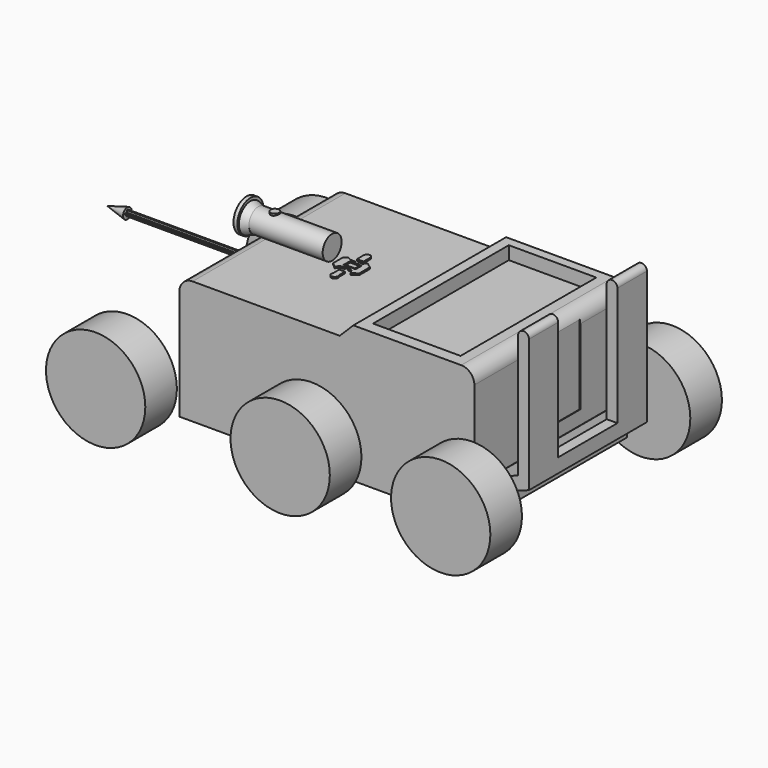
from build123d import *

# Parameters (mm, degrees)
F0_W           = 112
F0_H           = 52
F1_DEPTH       = 36.25
F1_DEPTH_BACK  = 36.25
F2_W           = 62.7835113555
F2_H           = 8.2989688963
F3_DEPTH       = 40
F3_DEPTH_BACK  = 40
F4_SIZE        = 5
F5_R           = 5
F8_DEPTH       = 0.6
F9_W           = 3.3755060285
F9_H           = 2.0101326518
F10_DEPTH      = 0.6
F12_R          = 18.8548205179
F13_DEPTH      = 15
F19_R          = 18.8548205179
F20_DEPTH      = 15
F24_DEPTH      = 28
F24_DEPTH_BACK = 28
F26_W          = 28.1342324962
F26_H          = 48.9349166028
F27_DEPTH      = 25
F29_R          = 4.5035590708
F30_DEPTH      = 28
F32_R          = 6.2065419795
F33_DEPTH      = 1.5
F36_R          = 4.4303853292
F37_DEPTH      = 25
F38_R          = 1.617072427
F39_DEPTH      = 9.3
F40_W          = 33.2386381924
F40_H          = 64.4318200648
F41_DEPTH      = 25
F42_R          = 1.0614733058
F43_DEPTH      = 80
F45_DEPTH      = 90


# Not quite as in the source:
# - the program builds the solid bodies; features that only make, move or delete a surface that nothing else refers to are left out


with BuildPart() as f1:
    # F0 (on Front) → F1 (new body, two sides)
    with BuildSketch(Plane.XZ) as f1_sk:
        Rectangle(F0_W, F0_H)
    extrude(amount=F1_DEPTH)
    extrude(f1_sk.sketch, amount=-F1_DEPTH_BACK)

    # F2 (on Front) → F3 (cut, two sides)
    with BuildSketch(Plane.XZ) as f3_sk:
        with Locations((-26.3402080163, 24.9871136621)):
            Rectangle(F2_W, F2_H)
    extrude(amount=-F3_DEPTH, mode=Mode.SUBTRACT)
    extrude(f3_sk.sketch, amount=F3_DEPTH_BACK, mode=Mode.SUBTRACT)

    # F4
    f4_edges = [f1.edges().sort_by_distance(p)[0] for p in [
        (5.051548, 0, 26),
    ]]
    chamfer(f4_edges, length=F4_SIZE)

    # F5
    f5_edges = [f1.edges().sort_by_distance(p)[0] for p in [
        (56, 0, 26),
        (-56, 0, 20.837629),
    ]]
    fillet(f5_edges, radius=F5_R)

    # F23 (on Front) → F24 (join, two sides)
    with BuildSketch(Plane.XZ) as f24_sk:
        with BuildLine():
            Line((66.0493522882, -9.3606118894), (56.0777671635, -12.9401576556))
            ThreePointArc((56.0777671635, -12.9401576556), (52.810402565, -15.2911024559), (56.0777671635, -17.6420472562))
            Line((56.0777671635, -17.6420472562), (70.1072718896, -12.9401576556))
            Line((70.1072718896, -12.9401576556), (70.1072718896, 37.5393816017))
            ThreePointArc((70.1072718896, 37.5393816017), (67.878123137, 39.5765729642), (66.0493522882, 37.1734812074))
            Line((66.0493522882, 37.1734812074), (66.0493522882, -9.3606118894))
        make_face()
    extrude(amount=F24_DEPTH)
    extrude(f24_sk.sketch, amount=-F24_DEPTH_BACK)

    # F26 (on offset) → F27 (cut)
    with BuildSketch(Plane.YZ.offset(55.8)):
        with Locations((-0.0549908727, 16.8750025332)):
            Rectangle(F26_W, F26_H)
    extrude(amount=F27_DEPTH, mode=Mode.SUBTRACT)

    # F29 (on offset) → F30 (join)
    with BuildSketch(Plane.YZ.offset(-27)):
        with Locations((0, 25.3125000745)):
            Circle(F29_R)
    extrude(amount=-F30_DEPTH)

    # F38 (on offset) → F39 (join)
    with BuildSketch(Plane.XY.offset(21)):
        with Locations((-48.7517826259, 0)):
            Circle(F38_R)
    extrude(amount=F39_DEPTH)

    # F40 (on offset) → F41 (cut)
    with BuildSketch(Plane.XY.offset(21)):
        with Locations((30.5095855147, 0.5113650113)):
            Rectangle(F40_W, F40_H)
    extrude(amount=F41_DEPTH, mode=Mode.SUBTRACT)

    # F42 (on offset) → F43 (join)
    with BuildSketch(Plane.YZ.offset(-27)):
        with Locations((0, 11.5056820214)):
            Circle(F42_R)
    extrude(amount=-F43_DEPTH)

    # F44 (on offset) → F45 (cut)
    with BuildSketch(Plane.YZ.offset(-58)):
        Polygon((-0.9458741988, 10.3932730854), (-0.3025215992, 10.4609942064), (-0.3025215992, 11.1382082105), (-1.1828994611, 11.1382082105), align=None)
        Polygon((1.2212089496, 11.1382082105), (0.3069706145, 11.1382082105), (0.3069706145, 10.4609942064), (0.8487420273, 10.3594120592), align=None)
        Polygon((-1.3505744282, 11.729169637), (-0.2593955433, 11.729169637), (-0.2593955433, 12.6839512959), (-1.2141767656, 12.4306418002), (-1.2921184534, 12.0214503258), (-1.3505744282, 11.865567416), align=None)
        Polygon((1.1240632739, 12.7813778818), (0.3056792775, 12.7813778818), (0.3056792775, 11.7486547679), (1.2604609365, 11.7486547679), align=None)
    extrude(amount=-F45_DEPTH, mode=Mode.SUBTRACT)

    # F46 (on Front) → F47 (revolve)
    with BuildSketch(Plane.XZ):
        Polygon((-104.7758087516, 9.3221208081), (-104.7758087516, 11.3514680415), (-112.3858690262, 11.3514680415), align=None)
    revolve(axis=Axis((-108.5808388889, 0, 11.3514680415), (1, 0, 0)))


with BuildPart() as f8:
    # F7 (on offset) → F8 (new body)
    with BuildSketch(Plane.XY.offset(21)):
        Polygon((-14.7115389197, -2.5), (-14.7115389197, 0), (-14.7115389197, 2.5), (-16.7638007551, 4.1132308543), (-17.7618643205, 2.8435503501), (-19.036853686, 2.8435503501), (-19.036853686, 1.7265254864), (-17.2184109688, 1.7265254864), (-17.2184109688, -1.1147919577), (-19.150506705, -1.1147919577), (-19.150506705, -2.2513177246), (-17.7866742015, -2.2513177246), (-16.8774537742, -3.9561078884), align=None)
    extrude(amount=F8_DEPTH)


with BuildPart() as f8b:
    # F7 (on offset) → F8, piece 2 (new body)
    with BuildSketch(Plane.XY.offset(21)):
        Polygon((-21.7645186931, 1.7265254864), (-20.2870331705, 1.7265254864), (-20.2870331705, 2.63574766), (-22.4464330822, 2.7494002134), (-23.6966125667, 3.5449680872), (-24.8860276497, 2.1811358165), (-24.8860276497, -2.1770501812), (-23.1283511966, -3.6151502281), (-22.1054758877, -2.364970278), (-20.5143392086, -2.1376651712), (-20.2870331705, -1.2284446275), (-21.7645186931, -1.2284446275), align=None)
    extrude(amount=F8_DEPTH)


with BuildPart() as f8c:
    # F7 (on offset) → F8, piece 3 (new body)
    with BuildSketch(Plane.XY.offset(21)):
        with BuildLine():
            Line((-18.6958964914, -7.1383831091), (-18.6958964914, -4.2970655486))
            Line((-18.6958964914, -4.2970655486), (-20.8552982658, -4.2970655486))
            Line((-20.8552982658, -4.2970655486), (-20.8552982658, -7.1383831091))
            ThreePointArc((-20.8552982658, -7.1383831091), (-19.7755973786, -9.0647520211), (-18.6958964914, -7.1383831091))
        make_face()
    extrude(amount=F8_DEPTH)


with BuildPart() as f8d:
    # F7 (on offset) → F8, piece 4 (new body)
    with BuildSketch(Plane.XY.offset(21)):
        with BuildLine():
            Line((-20.9689494222, 4.2268852703), (-18.4685904533, 4.2268852703))
            Line((-18.4685904533, 4.2268852703), (-18.4685904533, 7.4091586284))
            ThreePointArc((-18.4685904533, 7.4091586284), (-19.7187699378, 8.6593381129), (-20.9689494222, 7.4091586284))
            Line((-20.9689494222, 7.4091586284), (-20.9689494222, 4.2268852703))
        make_face()
    extrude(amount=F8_DEPTH)


with BuildPart() as f10:
    # F9 (on offset) → F10 (new body)
    with BuildSketch(Plane.XY.offset(21)):
        with Locations((-19.4186167791, 0.2163989702)):
            Rectangle(F9_W, F9_H)
    extrude(amount=F10_DEPTH)


with BuildPart() as f13:
    # F12 (on offset) → F13 (new body)
    with BuildSketch(Plane.XZ.offset(40)):
        with Locations((-72.8026961442, -14.5231969655)):
            Circle(F12_R)
    extrude(amount=F13_DEPTH)


with BuildPart() as f13b:
    # F12 (on offset) → F13, piece 2 (new body)
    with BuildSketch(Plane.XZ.offset(40)):
        with Locations((-2.735605929, -14.5231969655)):
            Circle(F12_R)
    extrude(amount=F13_DEPTH)


with BuildPart() as f13c:
    # F12 (on offset) → F13, piece 3 (new body)
    with BuildSketch(Plane.XZ.offset(40)):
        with Locations((58.2187140826, -14.5231969655)):
            Circle(F12_R)
    extrude(amount=F13_DEPTH)


with BuildPart() as f20:
    # F19 (on offset) → F20 (new body)
    with BuildSketch(Plane.XZ.offset(-40)):
        with Locations((-72.8781877551, -14.3427830189)):
            Circle(F19_R)
    extrude(amount=-F20_DEPTH)


with BuildPart() as f20b:
    # F19 (on offset) → F20, piece 2 (new body)
    with BuildSketch(Plane.XZ.offset(-40)):
        with Locations((-2.81109754, -14.3427830189)):
            Circle(F19_R)
    extrude(amount=-F20_DEPTH)


with BuildPart() as f20c:
    # F19 (on offset) → F20, piece 3 (new body)
    with BuildSketch(Plane.XZ.offset(-40)):
        with Locations((58.1432224717, -14.3427830189)):
            Circle(F19_R)
    extrude(amount=-F20_DEPTH)


with BuildPart() as f33:
    # F32 (on offset) → F33 (new body)
    with BuildSketch(Plane.YZ.offset(-58)):
        with Locations((0, 25.5681835115)):
            Circle(F32_R)
    extrude(amount=-F33_DEPTH)


with BuildPart() as f35:
    # F34 (on Front) → F35 (revolve)
    with BuildSketch(Plane.XZ):
        Polygon((-58.1059716642, 19.5757467947), (-55.047005415, 20.6966028265), (-55.116587552, 25.1466028265), (-58.1059716642, 25.1466028265), align=None)
    revolve(axis=Axis((-56.6112796081, 0, 25.1466028265), (1, 0, 0)))


with BuildPart() as f37_tool:
    # F36 (on offset) → F37 (new body)
    with BuildSketch(Plane.YZ.offset(-58)):
        with Locations((0, 25.3125000745)):
            Circle(F36_R)
    extrude(amount=-F37_DEPTH)


with BuildPart() as f33_1:
    add(f33.part)

    # F37: cut by f37_tool
    add(f37_tool.part, mode=Mode.SUBTRACT)


with BuildPart() as f35_1:
    add(f35.part)

    # F37: cut by f37_tool
    add(f37_tool.part, mode=Mode.SUBTRACT)


solid = Compound([f1.part, f8.part, f8b.part, f8c.part, f8d.part, f10.part, f13.part, f13b.part, f13c.part, f20.part, f20b.part, f20c.part, f33_1.part, f35_1.part])
